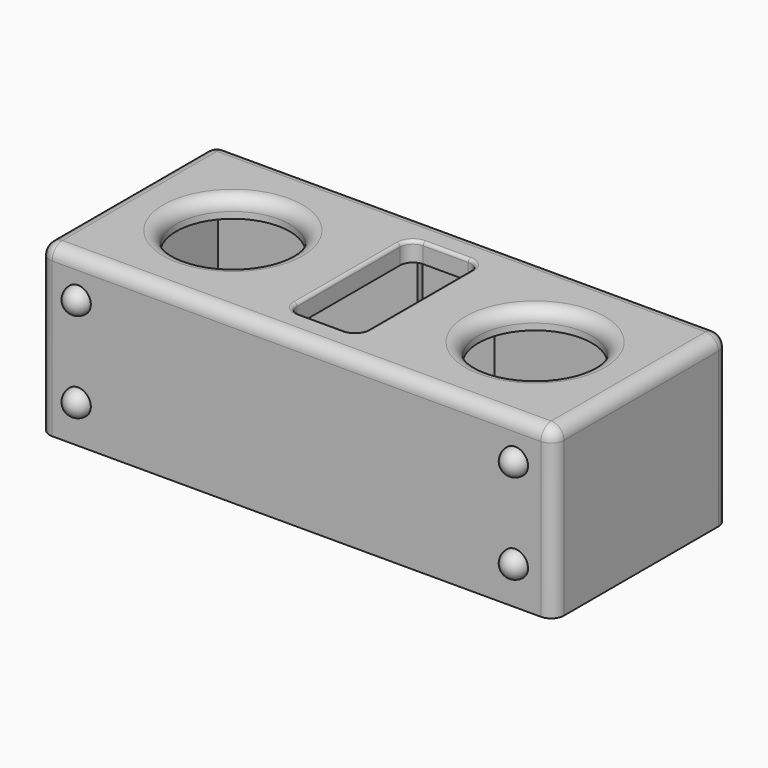
from build123d import *

# Parameters (mm, degrees)
F0_W     = 508
F0_H     = 215.9
F1_DEPTH = 165.1
F0_W_2   = 196.85
F0_H_2   = 177.8
F0_R     = 56
F0_W_3   = 76.2
F2_DEPTH = 19.05
F4_DEPTH = 146.05
F5_R     = 12.7
F6_R     = 3.175
F7_R     = 12.7
F8_DEPTH = 12.7
F9_R     = 12.69999
F10_R    = 12.7


# Not quite as in the source:
# - a fillet or chamfer is up to 0.001 mm smaller than in the source, because OpenCascade refuses the exact size


with BuildPart() as f1:
    # F0 (on Top) → F1 (new body)
    with BuildSketch(Plane.XY):
        Rectangle(F0_W, F0_H)
        Polygon((234.95, -88.9), (38.1, -88.9), (-38.1, -88.9), (-234.95, -88.9), (-234.95, 88.9), (-38.1, 88.9), (38.1, 88.9), (234.95, 88.9), align=None, mode=Mode.SUBTRACT)
    extrude(amount=-F1_DEPTH)

    # F0 (on Top) → F2 (join)
    with BuildSketch(Plane.XY):
        with Locations((-136.525, 0)):
            Rectangle(F0_W_2, F0_H_2)
        with Locations((-149.225, 0)):
            Circle(F0_R, mode=Mode.SUBTRACT)
        with Locations((136.525, 0)):
            Rectangle(F0_W_2, F0_H_2)
        with Locations((149.225, 0)):
            Circle(F0_R, mode=Mode.SUBTRACT)
        Rectangle(F0_W_3, F0_H_2)
        with BuildLine():
            ThreePointArc((34.925, -63.5), (31.2052561211, -72.4802561211), (22.225, -76.2))
            Line((22.225, -76.2), (-22.225, -76.2))
            ThreePointArc((-22.225, -76.2), (-31.2052561211, -72.4802561211), (-34.925, -63.5))
            Line((-34.925, -63.5), (-34.925, 63.5))
            ThreePointArc((-34.925, 63.5), (-31.2052561211, 72.4802561211), (-22.225, 76.2))
            Line((-22.225, 76.2), (22.225, 76.2))
            ThreePointArc((22.225, 76.2), (31.2052561211, 72.4802561211), (34.925, 63.5))
            Line((34.925, 63.5), (34.925, -63.5))
        make_face(mode=Mode.SUBTRACT)
    extrude(amount=-F2_DEPTH)

    # F3 (on face) → F4 (cut)
    with BuildSketch(Plane(origin=(0, 0, -165.1), x_dir=(1, 0, 0), z_dir=(0, 0, -1))):
        Polygon((-38.1, -88.9), (0, -88.9), (38.1, -88.9), (234.95, -88.9), (234.95, 88.9), (38.1, 88.9), (0, 88.9), (-38.1, 88.9), (-234.95, 88.9), (-234.95, -88.9), align=None)
        Polygon((38.1, -88.9), (0, -88.9), (-38.1, -88.9), (-38.1, -95.25), (38.1, -95.25), align=None)
        Polygon((0, 88.9), (38.1, 88.9), (38.1, 95.25), (-38.1, 95.25), (-38.1, 88.9), align=None)
    extrude(amount=-F4_DEPTH, mode=Mode.SUBTRACT)

    # F5
    f5_edges = [f1.edges().sort_by_distance(p)[0] for p in [
        (93.225, 0, 0),
        (-205.225, 0, 0),
    ]]
    fillet(f5_edges, radius=F5_R)

    # F6
    f6_edges = [f1.edges().sort_by_distance(p)[0] for p in [
        (0, 76.2, 0),
        (-34.925, 0, 0),
        (-31.205256, 72.480256, 0),
        (31.205256, 72.480256, 0),
        (34.925, 0, 0),
        (31.205256, -72.480256, 0),
        (0, -76.2, 0),
        (-31.205256, -72.480256, 0),
    ]]
    fillet(f6_edges, radius=F6_R)

    # F7 (on face) → F8 (join)
    with BuildSketch(Plane.XZ.offset(107.95)):
        with Locations((-215.9, -38.1)):
            Circle(F7_R)
        with Locations((-215.9, -127)):
            Circle(F7_R)
        with Locations((215.9, -38.1)):
            Circle(F7_R)
        with Locations((215.9, -127)):
            Circle(F7_R)
    extrude(amount=F8_DEPTH)

    # F9 (radius 12.7 in the source; OpenCascade refuses exactly that, so slightly less here)
    f9_edges = [f1.edges().sort_by_distance(p)[0] for p in [
        (-228.6, -120.65, -127),
        (-228.6, -120.65, -38.1),
        (203.2, -120.65, -38.1),
        (203.2, -120.65, -127),
    ]]
    fillet(f9_edges, radius=F9_R)

    # F10
    f10_edges = [f1.edges().sort_by_distance(p)[0] for p in [
        (254, 107.95, -82.55),
        (254, -107.95, -82.55),
        (-254, -107.95, -82.55),
        (-254, 107.95, -82.55),
        (254, 0, 0),
        (0, 107.95, 0),
        (0, -107.95, 0),
        (-254, 0, 0),
    ]]
    fillet(f10_edges, radius=F10_R)


solid = f1.part
